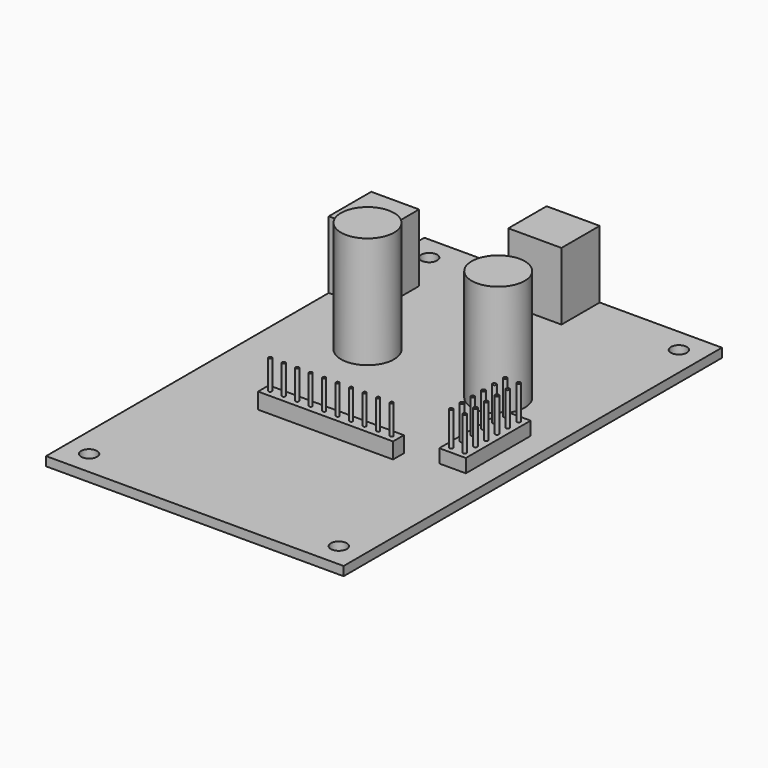
from build123d import *

# Parameters (mm, degrees)
F0_R     = 5
F1_DEPTH = 21
F0_R_2   = 1.5
F0_W     = 9
F0_H     = 10
F0_W_2   = 10
F0_H_2   = 9
F2_DEPTH = 1.7
F3_DEPTH = 12.7
F4_R     = 0.35
F5_DEPTH = 8.9
F4_W     = 5
F4_H     = 2.54
F6_DEPTH = 2.54
F4_R_2   = 0.3
F7_DEPTH = 8.5
F4_W_2   = 2.54
F8_DEPTH = 3


# Not quite as in the source:
# - a feature names something its author has since deleted; it is built from what else it names


with BuildPart() as f1:
    # F0 (on Top) → F1 (new body)
    with BuildSketch(Plane.XY):
        with Locations((12.3, 11.5)):
            Circle(F0_R)
    extrude(amount=F1_DEPTH)


with BuildPart() as f1b:
    # F0 (on Top) → F1, piece 2 (new body)
    with BuildSketch(Plane.XY):
        with Locations((-12.3, 11.5)):
            Circle(F0_R)
    extrude(amount=F1_DEPTH)


with BuildPart() as f2:
    # F0 (on Top) → F2 (new body)
    with BuildSketch(Plane.XY):
        Polygon((-28, -44.5), (28, -44.5), (28, 44.5), (5, 44.5), (5, 35.5), (-5, 35.5), (-5, 44.5), (-28, 44.5), (-28, 32), (-19, 32), (-19, 22), (-28, 22), align=None)
        with Locations((-23.5, -40)):
            Circle(F0_R_2, mode=Mode.SUBTRACT)
        with Locations((23.5, -40)):
            Circle(F0_R_2, mode=Mode.SUBTRACT)
        with Locations((-12.3, 11.5)):
            Circle(F0_R, mode=Mode.SUBTRACT)
        with Locations((-23.5, 40)):
            Circle(F0_R_2, mode=Mode.SUBTRACT)
        with Locations((12.3, 11.5)):
            Circle(F0_R, mode=Mode.SUBTRACT)
        with Locations((23.5, 40)):
            Circle(F0_R_2, mode=Mode.SUBTRACT)
        with Locations((-23.5, 27)):
            Rectangle(F0_W, F0_H)
        with Locations((0, 40)):
            Rectangle(F0_W_2, F0_H_2)
        with Locations((12.3, 11.5)):
            Circle(F0_R)
        with Locations((-12.3, 11.5)):
            Circle(F0_R)
    extrude(amount=-F2_DEPTH)

    # F0 (on Top) → F3 (join)
    with BuildSketch(Plane.XY):
        with Locations((0, 40)):
            Rectangle(F0_W_2, F0_H_2)
        with Locations((-23.5, 27)):
            Rectangle(F0_W, F0_H)
    extrude(amount=F3_DEPTH)

    # F4 (on face) → F5 (join)
    with BuildSketch(Plane.XY):
        with Locations((19.83, -6.44)):
            Circle(F4_R)
        with Locations((22.37, -6.44)):
            Circle(F4_R)
        with Locations((22.37, -8.98)):
            Circle(F4_R)
        with Locations((19.83, -8.98)):
            Circle(F4_R)
        with Locations((19.83, -3.9)):
            Circle(F4_R)
        with Locations((22.37, -3.9)):
            Circle(F4_R)
        with Locations((19.83, 1.18)):
            Circle(F4_R)
        with Locations((19.83, -1.36)):
            Circle(F4_R)
        with Locations((22.37, -1.36)):
            Circle(F4_R)
        with Locations((22.37, 1.18)):
            Circle(F4_R)
        with Locations((22.37, 3.72)):
            Circle(F4_R)
        with Locations((19.83, 3.72)):
            Circle(F4_R)
    extrude(amount=F5_DEPTH)

    # F4 (on face) → F6 (join)
    with BuildSketch(Plane.XY):
        with Locations((21.1, -1.36)):
            Rectangle(F4_W, F4_H)
        with Locations((19.83, -1.36)):
            Circle(F4_R, mode=Mode.SUBTRACT)
        with Locations((22.37, -1.36)):
            Circle(F4_R, mode=Mode.SUBTRACT)
        with Locations((21.1, -3.9)):
            Rectangle(F4_W, F4_H)
        with Locations((19.83, -3.9)):
            Circle(F4_R, mode=Mode.SUBTRACT)
        with Locations((22.37, -3.9)):
            Circle(F4_R, mode=Mode.SUBTRACT)
        with Locations((21.1, -6.44)):
            Rectangle(F4_W, F4_H)
        with Locations((19.83, -6.44)):
            Circle(F4_R, mode=Mode.SUBTRACT)
        with Locations((22.37, -6.44)):
            Circle(F4_R, mode=Mode.SUBTRACT)
        with Locations((21.1, 1.18)):
            Rectangle(F4_W, F4_H)
        with Locations((19.83, 1.18)):
            Circle(F4_R, mode=Mode.SUBTRACT)
        with Locations((22.37, 1.18)):
            Circle(F4_R, mode=Mode.SUBTRACT)
        with Locations((21.1, 3.72)):
            Rectangle(F4_W, F4_H)
        with Locations((19.83, 3.72)):
            Circle(F4_R, mode=Mode.SUBTRACT)
        with Locations((22.37, 3.72)):
            Circle(F4_R, mode=Mode.SUBTRACT)
        with Locations((21.1, -8.98)):
            Rectangle(F4_W, F4_H)
        with Locations((19.83, -8.98)):
            Circle(F4_R, mode=Mode.SUBTRACT)
        with Locations((22.37, -8.98)):
            Circle(F4_R, mode=Mode.SUBTRACT)
    extrude(amount=F6_DEPTH)

    # F4 (on face) → F7 (join)
    with BuildSketch(Plane.XY):
        with Locations((-11.63, -12.23)):
            Circle(F4_R_2)
        with Locations((-9.09, -12.23)):
            Circle(F4_R_2)
        with Locations((-6.55, -12.23)):
            Circle(F4_R_2)
        with Locations((-4.01, -12.23)):
            Circle(F4_R_2)
        with Locations((-1.47, -12.23)):
            Circle(F4_R_2)
        with Locations((1.07, -12.23)):
            Circle(F4_R_2)
        with Locations((3.61, -12.23)):
            Circle(F4_R_2)
        with Locations((6.15, -12.23)):
            Circle(F4_R_2)
        with Locations((8.69, -12.23)):
            Circle(F4_R_2)
        with Locations((11.23, -12.23)):
            Circle(F4_R_2)
    extrude(amount=F7_DEPTH)

    # F4 (on face) → F8 (join)
    with BuildSketch(Plane.XY):
        with Locations((-11.63, -12.23)):
            Rectangle(F4_W_2, F4_H)
        with Locations((-11.63, -12.23)):
            Circle(F4_R_2, mode=Mode.SUBTRACT)
        with Locations((-9.09, -12.23)):
            Rectangle(F4_W_2, F4_H)
        with Locations((-9.09, -12.23)):
            Circle(F4_R_2, mode=Mode.SUBTRACT)
        with Locations((-6.55, -12.23)):
            Rectangle(F4_W_2, F4_H)
        with Locations((-6.55, -12.23)):
            Circle(F4_R_2, mode=Mode.SUBTRACT)
        with Locations((-4.01, -12.23)):
            Rectangle(F4_W_2, F4_H)
        with Locations((-4.01, -12.23)):
            Circle(F4_R_2, mode=Mode.SUBTRACT)
        with Locations((-1.47, -12.23)):
            Rectangle(F4_W_2, F4_H)
        with Locations((-1.47, -12.23)):
            Circle(F4_R_2, mode=Mode.SUBTRACT)
        with Locations((1.07, -12.23)):
            Rectangle(F4_W_2, F4_H)
        with Locations((1.07, -12.23)):
            Circle(F4_R_2, mode=Mode.SUBTRACT)
        with Locations((3.61, -12.23)):
            Rectangle(F4_W_2, F4_H)
        with Locations((3.61, -12.23)):
            Circle(F4_R_2, mode=Mode.SUBTRACT)
        with Locations((6.15, -12.23)):
            Rectangle(F4_W_2, F4_H)
        with Locations((6.15, -12.23)):
            Circle(F4_R_2, mode=Mode.SUBTRACT)
        with Locations((8.69, -12.23)):
            Rectangle(F4_W_2, F4_H)
        with Locations((8.69, -12.23)):
            Circle(F4_R_2, mode=Mode.SUBTRACT)
        with Locations((11.23, -12.23)):
            Rectangle(F4_W_2, F4_H)
        with Locations((11.23, -12.23)):
            Circle(F4_R_2, mode=Mode.SUBTRACT)
    extrude(amount=F8_DEPTH)


solid = Compound([f1.part, f1b.part, f2.part])
